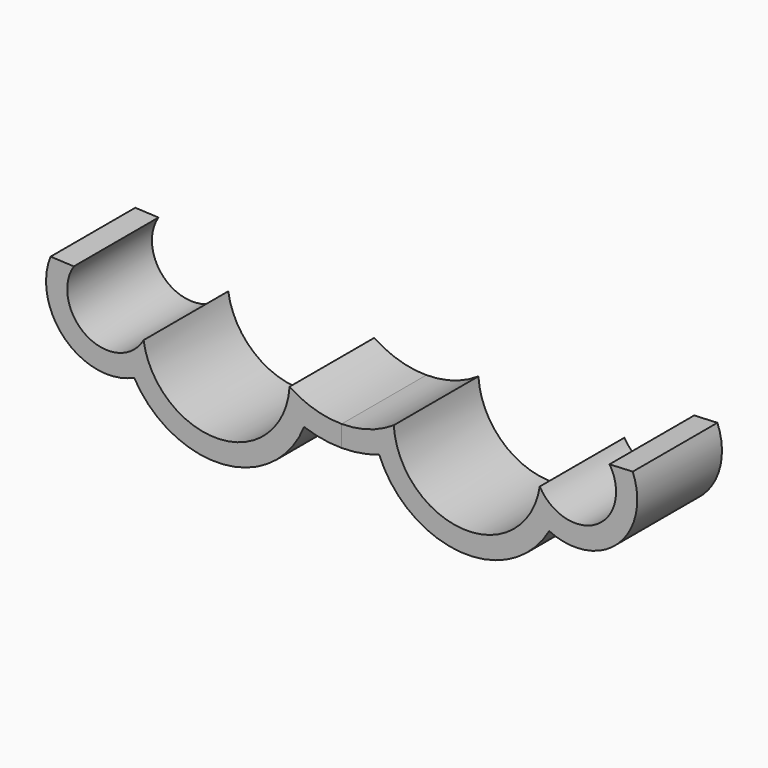
from build123d import *

# Parameters (mm, degrees)
F1_DEPTH = 100


# Not quite as in the source:
# - a pattern or mirror of a feature is missing from the dataset's text; its kind, count and spacing are read off the source's solid


with BuildPart() as f1:
    # F0 (on Front) → F1 (new body)
    with BuildSketch(Plane.XZ):
        with BuildLine():
            Line((-253.070826319, 15.4742012591), (-275, 16.4739655934))
            ThreePointArc((-275, 16.4739655934), (-261.0940304281, -47.9287208885), (-196.0785287696, -58.6089156394))
            ThreePointArc((-196.0785287696, -58.6089156394), (-112.2399003638, -103.305461967), (-35.4867419071, -47.3085912196))
            ThreePointArc((-35.4867419071, -47.3085912196), (-17.9923791465, -51.7727499469), (0, -53.2746601281))
            Line((0, -53.2746601281), (0, -33.2746601281))
            ThreePointArc((0, -33.2746601281), (-25.7203043518, -29.4557449875), (-49.2214237237, -18.3285010758))
            ThreePointArc((-49.2214237237, -18.3285010758), (-115.4421026575, -83.4579108167), (-187.166437391, -24.4440299182))
            ThreePointArc((-187.166437391, -24.4440299182), (-240.7101933499, -38.4812673083), (-253.070826319, 15.4742012591))
        make_face()
    extrude(amount=F1_DEPTH)


with BuildPart() as f1_copies_1:
    # F1_copies: instance of F1
    add(f1.part.mirror(Plane(origin=(0, 0, 0), x_dir=(0, 0, 1), z_dir=(1, 0, 0))))


solid = Compound([f1.part, f1_copies_1.part])
